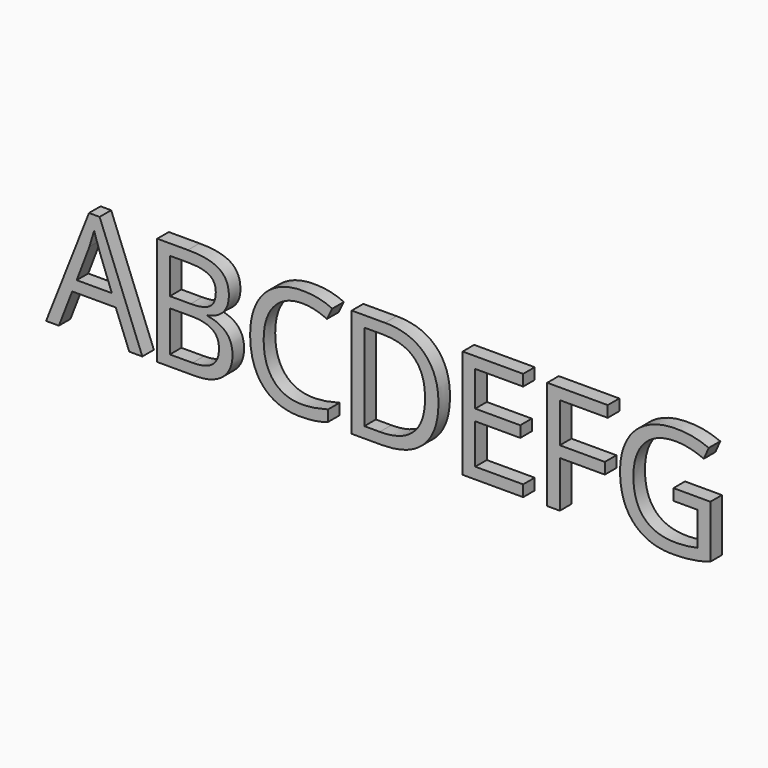
from build123d import *

# Parameters (mm, degrees)
F0_TEXT_SIZE = 31.5837710177
F1_DEPTH     = 3


# Not quite as in the source:
# - Text() gives the source's letters only with a copy of the font that has no kerning and outlines rounded to 1/6400 em; it was checked with that copy


with BuildPart() as f1:
    # F0 (on Front) → F1 (new body)
    with BuildSketch(Plane.XZ):
        with Locations((-70.8931648113, -10.1715837577)):
            Text('ABCDEFG', F0_TEXT_SIZE, font='Open Sans', text_align=(TextAlign.LEFT, TextAlign.BOTTOM))
    extrude(amount=F1_DEPTH)


solid = f1.part
